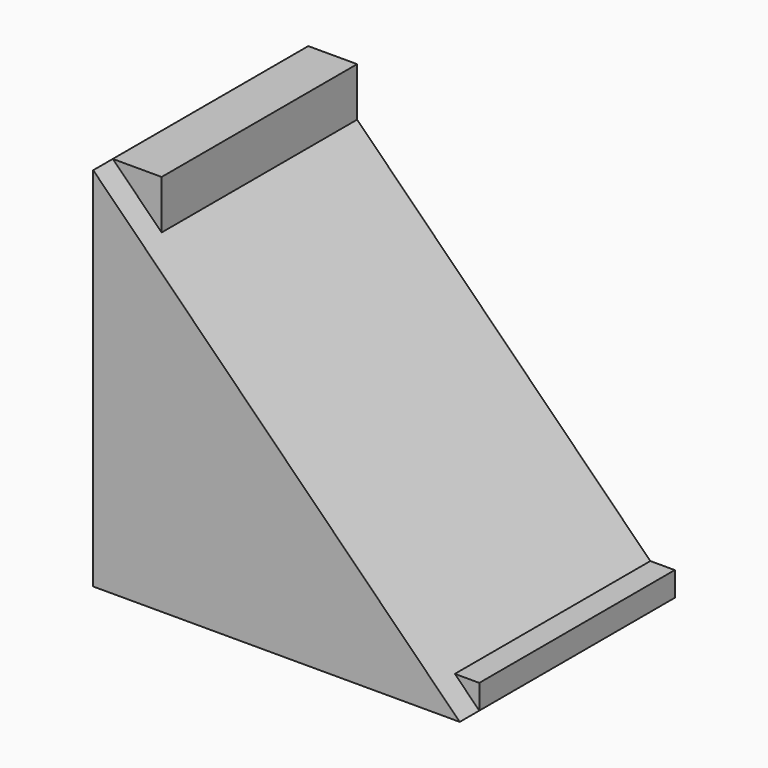
from build123d import *

# Parameters (mm, degrees)
F1_W     = 20
F1_H     = 30
F2_DEPTH = 4
F4_DEPTH = 2
F5_E7_W  = 30
F5_E7_H  = 20
F6_DEPTH = 2
F7_DEPTH = 20


with BuildPart() as f2:
    # F1 (on Right) → F2 (new body)
    with BuildSketch(Plane.YZ):
        with Locations((10, 15)):
            Rectangle(F1_W, F1_H)
    extrude(amount=F2_DEPTH)

    # F0 (on Front) → F4 (join)
    with BuildSketch(Plane.XZ):
        Polygon((0, 30), (0, 0), (30, 0), align=None)
    extrude(amount=F4_DEPTH)

    # F5_E7 (on explicit) → F6 (join)
    with BuildSketch(Plane.XY):
        with Locations((15, 10)):
            Rectangle(F5_E7_W, F5_E7_H)
    extrude(amount=F6_DEPTH)

    # F7 (add): a face of the model
    f7_faces = [f2.faces().sort_by_distance(p)[0] for p in [
        (12, 0, 10),
    ]]
    extrude(f7_faces, amount=F7_DEPTH)


solid = f2.part
